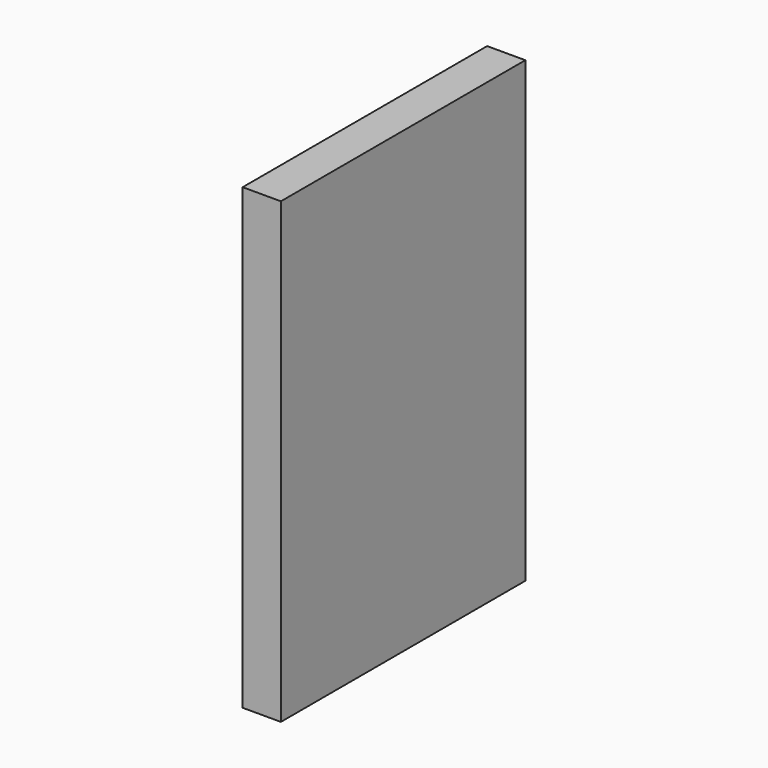
from build123d import *

# Parameters (mm, degrees)
F0_W     = 76.2
F0_H     = 114.3
F1_DEPTH = 9.525


# Not quite as in the source:
# - a length typed as a fraction of an inch, garbled in the dataset ("3 / 203.2 mm" for 3/8 in), is restored


with BuildPart() as f1:
    # F0 (on Right) → F1 (new body)
    with BuildSketch(Plane.YZ):
        Rectangle(F0_W, F0_H)
    extrude(amount=F1_DEPTH)


solid = f1.part
